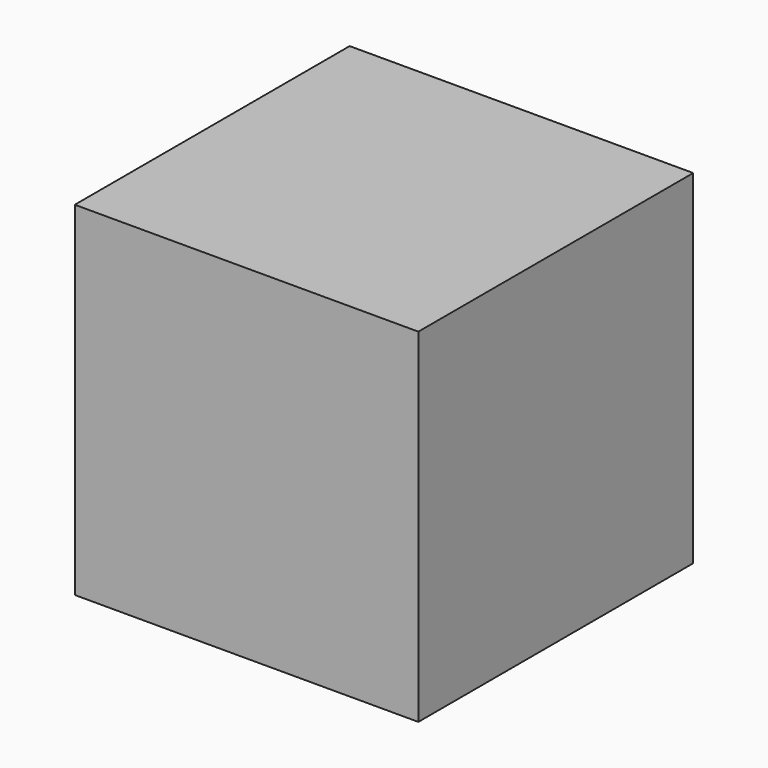
from build123d import *

# Parameters (mm, degrees)
F3_W     = 76.2
F3_H     = 76.2
F3_W_2   = 71.12
F3_H_2   = 71.12
F4_DEPTH = 38.1
F2_W     = 76.2
F2_H     = 76.2
F2_W_2   = 71.12
F2_H_2   = 71.12
F5_DEPTH = 38.1


# Not quite as in the source:
# - a variable given as a bare number and used for a length is read in inches; the dataset says mm whatever the document's units were


with BuildPart() as f4:
    # F3 (on Right) → F4 (new body, symmetric)
    with BuildSketch(Plane.YZ):
        Rectangle(F3_W, F3_H)
        Rectangle(F3_W_2, F3_H_2, mode=Mode.SUBTRACT)
    extrude(amount=F4_DEPTH, both=True)

    # F2 (on Front) → F5 (join, symmetric)
    with BuildSketch(Plane.XZ):
        Rectangle(F2_W, F2_H)
        Rectangle(F2_W_2, F2_H_2, mode=Mode.SUBTRACT)
    extrude(amount=F5_DEPTH, both=True)


solid = f4.part
